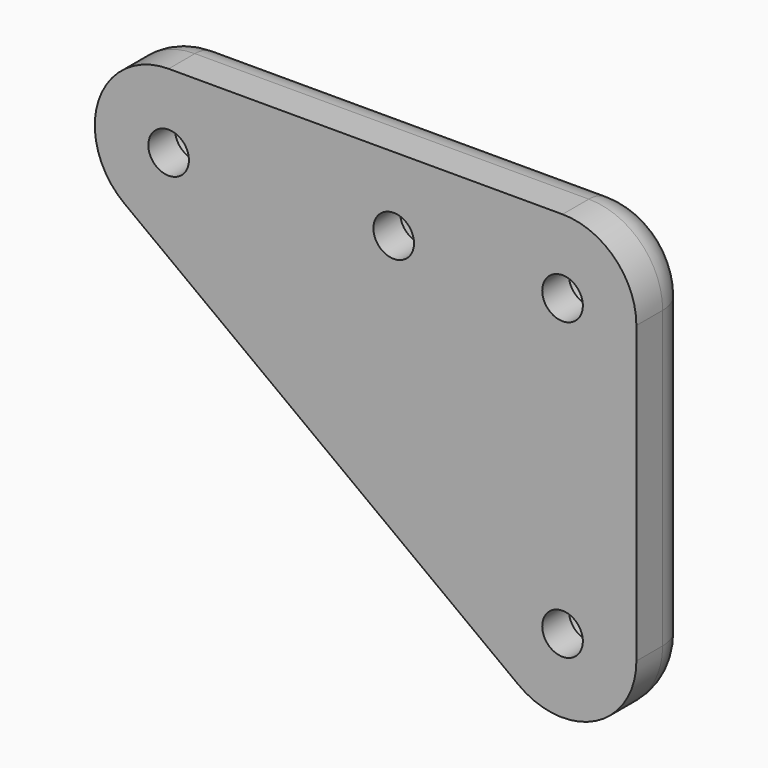
from build123d import *

# Parameters (mm, degrees)
F1_DEPTH       = 9.525
F2_D           = 5.5
F2_CBORE_D     = 9.75
F2_CBORE_DEPTH = 5
F3_R           = 5.08
F4_DEPTH       = 5
F5_D           = 5.5


# Not quite as in the source:
# - a feature names something its author has since deleted; it is built from what else it names


with BuildPart() as f1:
    # F0 (on Front) → F1 (new body)
    with BuildSketch(Plane.XZ):
        with BuildLine():
            Line((10, -40), (10, 0))
            ThreePointArc((10, 0), (7.0710678119, 7.0710678119), (0, 10))
            Line((0, 10), (-53.34, 10))
            ThreePointArc((-53.34, 10), (-62.826927837, 3.1619930765), (-59.3395200276, -8.0003599568))
            Line((-59.3395200276, -8.0003599568), (-5.9995200276, -48.0003599568))
            ThreePointArc((-5.9995200276, -48.0003599568), (4.4724042597, -48.9441377526), (10, -40))
        make_face()
        Polygon((-20.36, -4.1698729811), (-20.4062613559, -4.25), (-25.3137386441, -4.25), (-27.7674772881, 0), (-25.3137386441, 4.25), (-20.4062613559, 4.25), (-20.36, 4.1698729811), (-20.3137386441, 4.25), (-15.4062613559, 4.25), (-12.9525227119, 0), (-15.4062613559, -4.25), (-20.3137386441, -4.25), align=None, mode=Mode.SUBTRACT)
        Polygon((-25.3137386441, -4.25), (-20.4062613559, -4.25), (-20.36, -4.1698729811), (-22.7674772881, 0), (-20.36, 4.1698729811), (-20.4062613559, 4.25), (-25.3137386441, 4.25), (-27.7674772881, 0), align=None)
        Polygon((-17.9525227119, 0), (-20.36, -4.1698729811), (-20.3137386441, -4.25), (-15.4062613559, -4.25), (-12.9525227119, 0), (-15.4062613559, 4.25), (-20.3137386441, 4.25), (-20.36, 4.1698729811), align=None)
        Polygon((-22.7674772881, 0), (-20.36, -4.1698729811), (-17.9525227119, 0), (-20.36, 4.1698729811), align=None)
    extrude(amount=F1_DEPTH)

    # F2 (through all)
    with Locations(Plane(origin=(0, 0, 0), x_dir=(1, 0, 0), z_dir=(0, 1, 0))):
        with Locations((0, 0), (0, 40), (-53.34, 0)):
            CounterBoreHole(F2_D / 2, F2_CBORE_D / 2, F2_CBORE_DEPTH)

    # F3
    f3_edges = [f1.edges().sort_by_distance(p)[0] for p in [
        (-26.67, 0, 10),
    ]]
    fillet(f3_edges, radius=F3_R)

    # F0 (on Front) → F4 (cut)
    with BuildSketch(Plane.XZ):
        Polygon((-25.3137386441, -4.25), (-20.4062613559, -4.25), (-20.36, -4.1698729811), (-22.7674772881, 0), (-20.36, 4.1698729811), (-20.4062613559, 4.25), (-25.3137386441, 4.25), (-27.7674772881, 0), align=None)
        Polygon((-22.7674772881, 0), (-20.36, -4.1698729811), (-17.9525227119, 0), (-20.36, 4.1698729811), align=None)
        Polygon((-17.9525227119, 0), (-20.36, -4.1698729811), (-20.3137386441, -4.25), (-15.4062613559, -4.25), (-12.9525227119, 0), (-15.4062613559, 4.25), (-20.3137386441, 4.25), (-20.36, 4.1698729811), align=None)
    extrude(amount=F4_DEPTH, mode=Mode.SUBTRACT)

    # F5 (through all)
    with Locations(Plane(origin=(0, 0, 0), x_dir=(1, 0, 0), z_dir=(0, 1, 0))):
        with Locations((-22.86, 0)):
            Hole(F5_D / 2)


solid = f1.part
